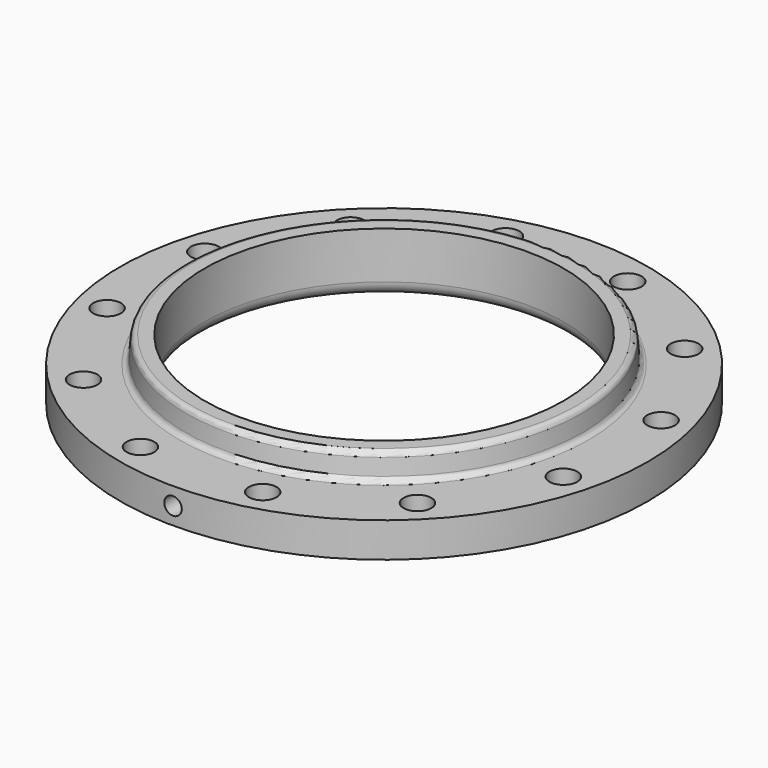
from build123d import *

# Parameters (mm, degrees)
F2_R     = 12.7
F3_DEPTH = 31.801
F4_R     = 8
F5_DEPTH = 241.301


# Not quite as in the source:
# - a feature names something its author has since deleted; it is built from what else it names


with BuildPart() as f1:
    # F0 (on Front) → F1 (revolve)
    with BuildSketch(Plane.XZ):
        with BuildLine():
            ThreePointArc((164.1, 12.7), (167.8197438789, 3.7197438789), (176.8, 0))
            Line((176.8, 0), (241.3, 0))
            Line((241.3, 0), (241.3, 31.8))
            Line((241.3, 31.8), (187.2316558701, 31.8))
            ThreePointArc((187.2316558701, 31.8), (183.853704832, 33.1136133159), (182.2506823796, 36.3642212863))
            Line((182.2506823796, 36.3642212863), (180.9670874285, 51.0357787137))
            ThreePointArc((180.9670874285, 51.0357787137), (179.3640649761, 54.2863866841), (175.986113938, 55.6))
            Line((175.986113938, 55.6), (164.1, 55.6))
            Line((164.1, 55.6), (164.1, 12.7))
        make_face()
    revolve(axis=Axis((0, 0, 27.8), (0, 0, 1)))

    # F2 (on face) → F3 (cut, through all)
    with BuildSketch(Plane.XY.offset(31.8)):
        with Locations((-55.8790318376, 208.5433858958)):
            Circle(F2_R)
        with Locations((-152.6643540582, 152.6643540582)):
            Circle(F2_R)
        with Locations((-208.5433858958, 55.8790318376)):
            Circle(F2_R)
        with Locations((-208.5433858958, -55.8790318376)):
            Circle(F2_R)
        with Locations((-152.6643540582, -152.6643540582)):
            Circle(F2_R)
        with Locations((-55.8790318376, -208.5433858958)):
            Circle(F2_R)
        with Locations((55.8790318376, -208.5433858958)):
            Circle(F2_R)
        with Locations((152.6643540582, -152.6643540582)):
            Circle(F2_R)
        with Locations((208.5433858958, -55.8790318376)):
            Circle(F2_R)
        with Locations((208.5433858958, 55.8790318376)):
            Circle(F2_R)
        with Locations((152.6643540582, 152.6643540582)):
            Circle(F2_R)
        with Locations((55.8790318376, 208.5433858958)):
            Circle(F2_R)
    extrude(amount=-F3_DEPTH, mode=Mode.SUBTRACT)

    # F4 (on Front) → F5 (cut, through all)
    with BuildSketch(Plane.XZ):
        with Locations((0, 15.9)):
            Circle(F4_R)
    extrude(amount=F5_DEPTH, mode=Mode.SUBTRACT)


solid = f1.part
